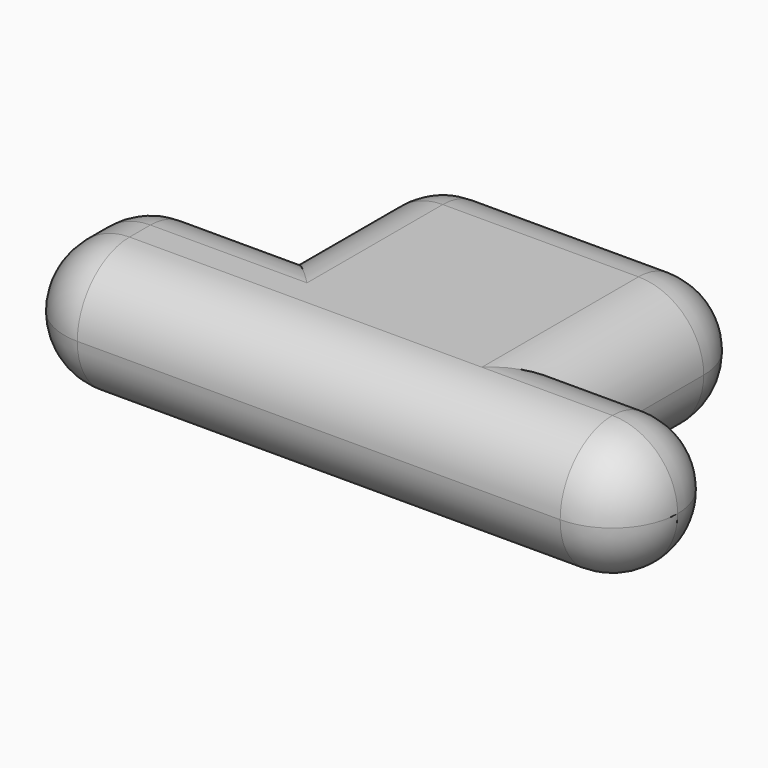
from build123d import *

# Parameters (mm, degrees)
F0_W     = 12
F0_H     = 12
F0_W_2   = 10
F0_H_2   = 10
F1_DEPTH = 10
F2_R     = 4.99999


# Not quite as in the source:
# - a fillet or chamfer is up to 0.001 mm smaller than in the source, because OpenCascade refuses the exact size


with BuildPart() as f1:
    # F0 (on Top) → F1 (new body)
    with BuildSketch(Plane.XY):
        Polygon((2.5256457627, 38.7224316552), (-22.4743542373, 38.7224316552), (-22.4743542373, 25.7224316552), (-22.4743542373, 13.7224316552), (2.5256457627, 13.7224316552), (2.5256457627, 23.7224316552), align=None)
        with Locations((-28.4743542373, 19.7224316552)):
            Rectangle(F0_W, F0_H)
        with Locations((7.5256457627, 18.7224316552)):
            Rectangle(F0_W_2, F0_H_2)
    extrude(amount=F1_DEPTH)

    # F2 (radius 5 in the source; OpenCascade refuses exactly that, so slightly less here)
    f2_edges = [f1.edges().sort_by_distance(p)[0] for p in [
        (-22.474354, 38.722432, 5),
        (-22.474354, 32.222432, 10),
        (-34.474354, 19.722432, 10),
        (-34.474354, 25.722432, 5),
        (-34.474354, 13.722432, 5),
        (-34.474354, 19.722432, 0),
        (2.525646, 31.222432, 10),
        (-9.974354, 38.722432, 10),
        (-28.474354, 25.722432, 10),
        (-10.974354, 13.722432, 10),
        (12.525646, 18.722432, 10),
        (7.525646, 23.722432, 10),
        (2.525646, 38.722432, 5),
        (-9.974354, 38.722432, 0),
        (7.525646, 23.722432, 0),
        (2.525646, 31.222432, 0),
        (-22.474354, 32.222432, 0),
        (-28.474354, 25.722432, 0),
        (-10.974354, 13.722432, 0),
        (12.525646, 18.722432, 0),
        (12.525646, 13.722432, 5),
        (12.525646, 23.722432, 5),
    ]]
    fillet(f2_edges, radius=F2_R)


solid = f1.part
